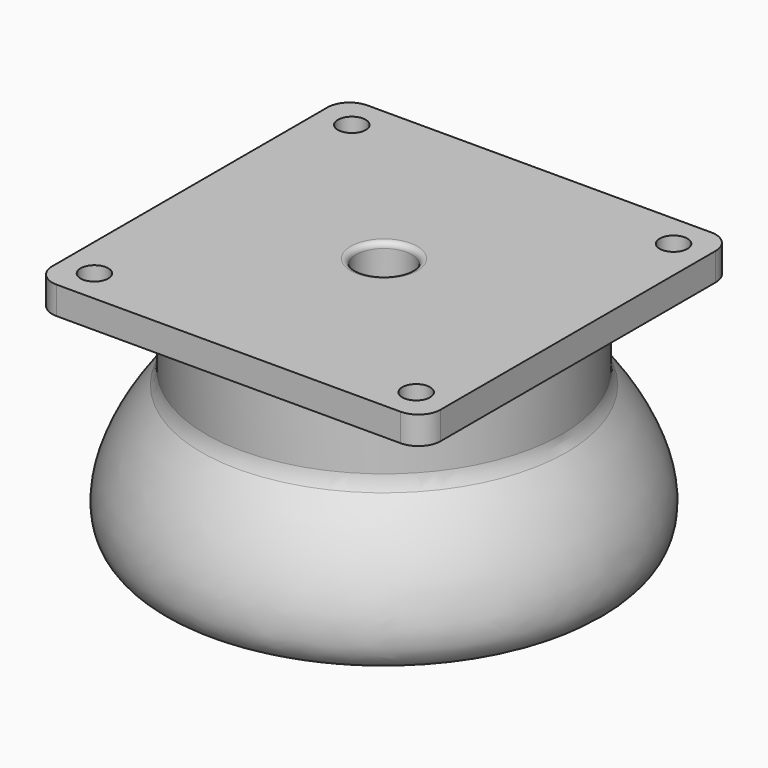
from build123d import *

# Parameters (mm, degrees)
F2_R     = 5.08
F3_R     = 3.175
F4_DEPTH = 6.35
F5_R     = 3.175
F6_DEPTH = 6.35
F7_R     = 5.08
F8_R     = 1.27


with BuildPart() as f1:
    # F0 (on Front) → F1 (revolve)
    with BuildSketch(Plane.XZ):
        with BuildLine():
            Line((61.3210011825, 30.4264344521), (10.5210011825, 30.4264344521))
            add(Edge.make_bspline(
                [(10.5210011825, 30.4264344521), (14.7434536794, 28.6604071042), (19.0713169557, 26.5881253305), (23.36869209, 24.0764344521)],
                knots=[0, 0, 0, 0, 0.0888010808, 0.0888010808, 0.0888010808, 0.0888010808], degree=3))
            Line((23.36869209, 24.0764344521), (35.9210011825, 24.0764344521))
            Line((35.9210011825, 24.0764344521), (44.8110011825, 24.0764344521))
            Line((44.8110011825, 24.0764344521), (61.3210011825, 24.0764344521))
            Line((61.3210011825, 24.0764344521), (61.3210011825, 30.4264344521))
        make_face()
        with BuildLine():
            Line((10.5210011825, 30.4264344521), (10.5210011825, 24.0764344521))
            Line((10.5210011825, 24.0764344521), (23.36869209, 24.0764344521))
            add(Edge.make_bspline(
                [(10.5210011825, 30.4264344521), (14.7434536794, 28.6604071042), (19.0713169557, 26.5881253305), (23.36869209, 24.0764344521)],
                knots=[0, 0, 0, 0, 0.0888010808, 0.0888010808, 0.0888010808, 0.0888010808], degree=3))
        make_face()
        with BuildLine():
            Line((35.9210011825, 24.0764344521), (23.36869209, 24.0764344521))
            add(Edge.make_bspline(
                [(23.36869209, 24.0764344521), (27.6267977125, 21.5876954621), (31.8549698498, 18.6675413362), (35.9210011825, 15.1864344521)],
                knots=[0.0888010808, 0.0888010808, 0.0888010808, 0.0888010808, 0.1767906953, 0.1767906953, 0.1767906953, 0.1767906953], degree=3))
            Line((35.9210011825, 15.1864344521), (35.9210011825, 24.0764344521))
        make_face()
        with BuildLine():
            Line((10.5210011825, 24.0764344521), (10.5210011825, 12.0998285711))
            add(Edge.make_bspline(
                [(44.8110011825, 6.3201577437), (49.5862497092, 0.7620105634), (57.5358513083, -11.7409030265), (57.0383379111, -28.1478545502), (38.5441102739, -28.0877230389), (38.3136411454, -10.3928004872), (25.344577473, 6.370842939), (14.8321684661, 9.5628876429), (10.5210011825, 12.0998285711)],
                knots=[0.2444339873, 0.2444339873, 0.2444339873, 0.2444339873, 0.3625729051, 0.4869256415, 0.5986829524, 0.7250488156, 0.8717448236, 1, 1, 1, 1], degree=3))
            add(Edge.make_bspline(
                [(35.9210011825, 15.1864344521), (39.046821731, 12.5102830554), (42.0768172491, 9.5026092192), (44.8110011825, 6.3201577437)],
                knots=[0.1767906953, 0.1767906953, 0.1767906953, 0.1767906953, 0.2444339873, 0.2444339873, 0.2444339873, 0.2444339873], degree=3))
            add(Edge.make_bspline(
                [(23.36869209, 24.0764344521), (27.6267977125, 21.5876954621), (31.8549698498, 18.6675413362), (35.9210011825, 15.1864344521)],
                knots=[0.0888010808, 0.0888010808, 0.0888010808, 0.0888010808, 0.1767906953, 0.1767906953, 0.1767906953, 0.1767906953], degree=3))
            Line((23.36869209, 24.0764344521), (10.5210011825, 24.0764344521))
        make_face()
        with BuildLine():
            add(Edge.make_bspline(
                [(35.9210011825, 15.1864344521), (39.046821731, 12.5102830554), (42.0768172491, 9.5026092192), (44.8110011825, 6.3201577437)],
                knots=[0.1767906953, 0.1767906953, 0.1767906953, 0.1767906953, 0.2444339873, 0.2444339873, 0.2444339873, 0.2444339873], degree=3))
            Line((44.8110011825, 6.3201577437), (44.8110011825, 24.0764344521))
            Line((44.8110011825, 24.0764344521), (35.9210011825, 24.0764344521))
            Line((35.9210011825, 24.0764344521), (35.9210011825, 15.1864344521))
        make_face()
    revolve(axis=Axis((4.1710011825, 0, 12.3320174103), (0, 0, -1)))

    # F2
    f2_edges = [f1.edges().sort_by_distance(p)[0] for p in [
        (-36.468999, 0, 6.320158),
    ]]
    fillet(f2_edges, radius=F2_R)

    # F3 (on face) → F4 (cut, through all)
    with BuildSketch(Plane.XY.offset(30.4264344521)):
        with Locations((41.0010011825, 36.83)):
            Circle(F3_R)
        with Locations((41.0010011825, -36.83)):
            Circle(F3_R)
        with Locations((-32.6589988175, -36.83)):
            Circle(F3_R)
        with Locations((-32.6589988175, 36.83)):
            Circle(F3_R)
        with BuildLine():
            ThreePointArc((40.0920256668, 44.45), (23.2210012001, 53.8815367202), (4.1710012198, 57.15))
            ThreePointArc((4.1710012198, 57.15), (-14.8789987999, 53.8815367326), (-31.7500233018, 44.45))
            Line((-31.7500233018, 44.45), (40.0920256668, 44.45))
        make_face()
        with BuildLine():
            ThreePointArc((-40.2789988175, 35.9210244843), (-49.7105354989, 19.0500001274), (-52.9789988175, 2.702e-07))
            ThreePointArc((-52.9789988175, 2.702e-07), (-49.710535589, -19.0499998726), (-40.2789988175, -35.9210244843))
            Line((-40.2789988175, -35.9210244843), (-40.2789988175, 35.9210244843))
        make_face()
        with BuildLine():
            ThreePointArc((48.6210011825, -35.9210244843), (58.0525379089, -19.05), (61.3210011825, 0))
            ThreePointArc((61.3210011825, 0), (58.0525379089, 19.05), (48.6210011825, 35.9210244843))
            Line((48.6210011825, 35.9210244843), (48.6210011825, -35.9210244843))
        make_face()
        with BuildLine():
            ThreePointArc((-31.7500233018, -44.45), (-14.8789988624, -53.8815367105), (4.1710010872, -57.15))
            ThreePointArc((4.1710010872, -57.15), (23.2210011376, -53.8815367423), (40.0920256668, -44.45))
            Line((40.0920256668, -44.45), (-31.7500233018, -44.45))
        make_face()
        with BuildLine():
            Line((48.6210011825, -44.45), (48.6210011825, -35.9210244843))
            ThreePointArc((48.6210011825, -35.9210244843), (44.5821537273, -40.4111525448), (40.0920256668, -44.45))
            Line((40.0920256668, -44.45), (48.6210011825, -44.45))
        make_face()
        with BuildLine():
            ThreePointArc((-31.7500233018, -44.45), (-36.2401513623, -40.4111525448), (-40.2789988175, -35.9210244843))
            Line((-40.2789988175, -35.9210244843), (-40.2789988175, -44.45))
            Line((-40.2789988175, -44.45), (-31.7500233018, -44.45))
        make_face()
        with BuildLine():
            Line((48.6210011825, 44.45), (40.0920256668, 44.45))
            ThreePointArc((40.0920256668, 44.45), (44.5821537273, 40.4111525448), (48.6210011825, 35.9210244843))
            Line((48.6210011825, 35.9210244843), (48.6210011825, 44.45))
        make_face()
    extrude(amount=-F4_DEPTH, mode=Mode.SUBTRACT)

    # F5
    f5_edges = [f1.edges().sort_by_distance(p)[0] for p in [
        (-2.178999, 0, 12.099829),
    ]]
    fillet(f5_edges, radius=F5_R)

    # F3 (on face) → F6 (join, through all)
    with BuildSketch(Plane.XY.offset(30.4264344521)):
        with BuildLine():
            ThreePointArc((-40.2789988175, 35.9210244843), (-36.2401513623, 40.4111525448), (-31.7500233018, 44.45))
            Line((-31.7500233018, 44.45), (-40.2789988175, 44.45))
            Line((-40.2789988175, 44.45), (-40.2789988175, 35.9210244843))
        make_face()
        with BuildLine():
            ThreePointArc((-31.7500233018, -44.45), (-36.2401513623, -40.4111525448), (-40.2789988175, -35.9210244843))
            Line((-40.2789988175, -35.9210244843), (-40.2789988175, -44.45))
            Line((-40.2789988175, -44.45), (-31.7500233018, -44.45))
        make_face()
        with BuildLine():
            Line((48.6210011825, -44.45), (48.6210011825, -35.9210244843))
            ThreePointArc((48.6210011825, -35.9210244843), (44.5821537273, -40.4111525448), (40.0920256668, -44.45))
            Line((40.0920256668, -44.45), (48.6210011825, -44.45))
        make_face()
        with BuildLine():
            Line((48.6210011825, 44.45), (40.0920256668, 44.45))
            ThreePointArc((40.0920256668, 44.45), (44.5821537273, 40.4111525448), (48.6210011825, 35.9210244843))
            Line((48.6210011825, 35.9210244843), (48.6210011825, 44.45))
        make_face()
    extrude(amount=-F6_DEPTH)

    # F7
    f7_edges = [f1.edges().sort_by_distance(p)[0] for p in [
        (-40.278999, 44.45, 27.251434),
        (48.621001, 44.45, 27.251434),
        (48.621001, -44.45, 27.251434),
        (-40.278999, -44.45, 27.251434),
    ]]
    fillet(f7_edges, radius=F7_R)

    # F8
    f8_edges = [f1.edges().sort_by_distance(p)[0] for p in [
        (-2.178999, 0, 30.426434),
    ]]
    fillet(f8_edges, radius=F8_R)


solid = f1.part
